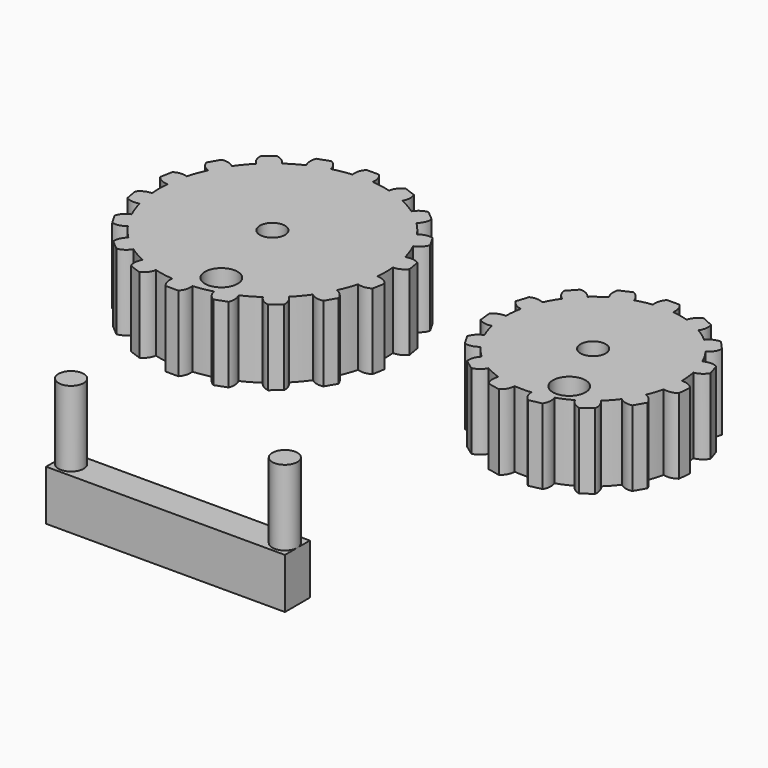
from build123d import *

# Parameters (mm, degrees)
F1_DEPTH  = 30
F0_R      = 6.5
F0_R_2    = 5
F2_DEPTH  = 30
F3_COUNT  = 18
F4_R      = 5
F4_R_2    = 6.5
F5_DEPTH  = 30
F6_DEPTH  = 30
F7_COUNT  = 15
F8_R      = 5
F9_DEPTH  = 20
F10_DEPTH = 30


with BuildPart() as f1:
    # F0 (on Top) → F1 (new body)
    with BuildSketch(Plane.XY):
        with BuildLine():
            ThreePointArc((-2.5, 49.9374608886), (-3.8493420396, 47.555405091), (-4, 44.821869662))
            Line((-4, 44.821869662), (4, 44.821869662))
            ThreePointArc((4, 44.821869662), (3.8493420396, 47.555405091), (2.5, 49.9374608886))
            Line((2.5, 49.9374608886), (-2.5, 49.9374608886))
        make_face()
    extrude(amount=F1_DEPTH)



with BuildPart() as f2:
    # F0 (on Top) → F2 (new body)
    with BuildSketch(Plane.XY):
        with BuildLine():
            Line((4, 44.821869662), (-4, 44.821869662))
            ThreePointArc((-4, 44.821869662), (0, -45), (4, 44.821869662))
        make_face()
        with Locations((7.5503932312, -34.8436161876)):
            Circle(F0_R, mode=Mode.SUBTRACT)
        Circle(F0_R_2, mode=Mode.SUBTRACT)
    extrude(amount=F2_DEPTH)


with BuildPart() as f1_1:
    add(f1.part)

    add(f2.part)  # F3 merges F2
    # F3: F1 ×18 about axis
    f3_axis = Axis((0, 0, 0), (0, 0, 1))
    for i in range(1, F3_COUNT):
        add(f1.part.rotate(f3_axis, i * 360 / F3_COUNT))


with BuildPart() as f5:
    # F4 (on Top) → F5 (new body)
    with BuildSketch(Plane.XY):
        with BuildLine():
            Line((131.5420866013, 34.7706773014), (123.5420866013, 34.7706773014))
            ThreePointArc((123.5420866013, 34.7706773014), (127.5420866013, -35), (131.5420866013, 34.7706773014))
        make_face()
        with Locations((127.5420866013, 0)):
            Circle(F4_R, mode=Mode.SUBTRACT)
        with Locations((137.5135779381, -24.3449360132)):
            Circle(F4_R_2, mode=Mode.SUBTRACT)
    extrude(amount=F5_DEPTH)



with BuildPart() as f6:
    # F4 (on Top) → F6 (new body)
    with BuildSketch(Plane.XY):
        with BuildLine():
            ThreePointArc((125.0420866013, 39.9217985567), (123.684267463, 37.523234094), (123.5420866013, 34.7706773014))
            Line((123.5420866013, 34.7706773014), (131.5420866013, 34.7706773014))
            ThreePointArc((131.5420866013, 34.7706773014), (131.3999057395, 37.523234094), (130.0420866013, 39.9217985567))
            Line((130.0420866013, 39.9217985567), (125.0420866013, 39.9217985567))
        make_face()
    extrude(amount=F6_DEPTH)


with BuildPart() as f5_1:
    add(f5.part)

    add(f6.part)  # F7 merges F6
    # F7: F6 ×15 about axis
    f7_axis = Axis((127.5420866013, 0, 0), (0, 0, 1))
    for i in range(1, F7_COUNT):
        add(f6.part.rotate(f7_axis, i * 360 / F7_COUNT))


with BuildPart() as f9:
    # F8 (on Top) → F9 (new body)
    with BuildSketch(Plane.XY):
        Polygon((103.4340906143, -110.6926842835), (8.4340906143, -110.6926842835), (8.4340906143, -116.8795691189), (8.4340906143, -123.0664581749), (103.4340906143, -123.0664581749), (103.4340906143, -116.8665662408), align=None)
        with BuildLine():
            ThreePointArc((18.4340906143, -116.8795691189), (13.4340906143, -121.8795691189), (8.4340906143, -116.8795691189))
            ThreePointArc((8.4340906143, -116.8795691189), (13.4340906143, -111.8795691189), (18.4340906143, -116.8795691189))
        make_face(mode=Mode.SUBTRACT)
        with Locations((98.4340906143, -116.8665662408)):
            Circle(F8_R, mode=Mode.SUBTRACT)
        with BuildLine():
            ThreePointArc((18.4340906143, -116.8795691189), (13.4340906143, -111.8795691189), (8.4340906143, -116.8795691189))
            ThreePointArc((8.4340906143, -116.8795691189), (13.4340906143, -121.8795691189), (18.4340906143, -116.8795691189))
        make_face()
        with Locations((98.4340906143, -116.8665662408)):
            Circle(F8_R)
    extrude(amount=-F9_DEPTH)

    # F8 (on Top) → F10 (join)
    with BuildSketch(Plane.XY):
        with Locations((98.4340906143, -116.8665662408)):
            Circle(F8_R)
        with BuildLine():
            ThreePointArc((18.4340906143, -116.8795691189), (13.4340906143, -111.8795691189), (8.4340906143, -116.8795691189))
            ThreePointArc((8.4340906143, -116.8795691189), (13.4340906143, -121.8795691189), (18.4340906143, -116.8795691189))
        make_face()
    extrude(amount=F10_DEPTH)


solid = Compound([f1_1.part, f5_1.part, f9.part])
